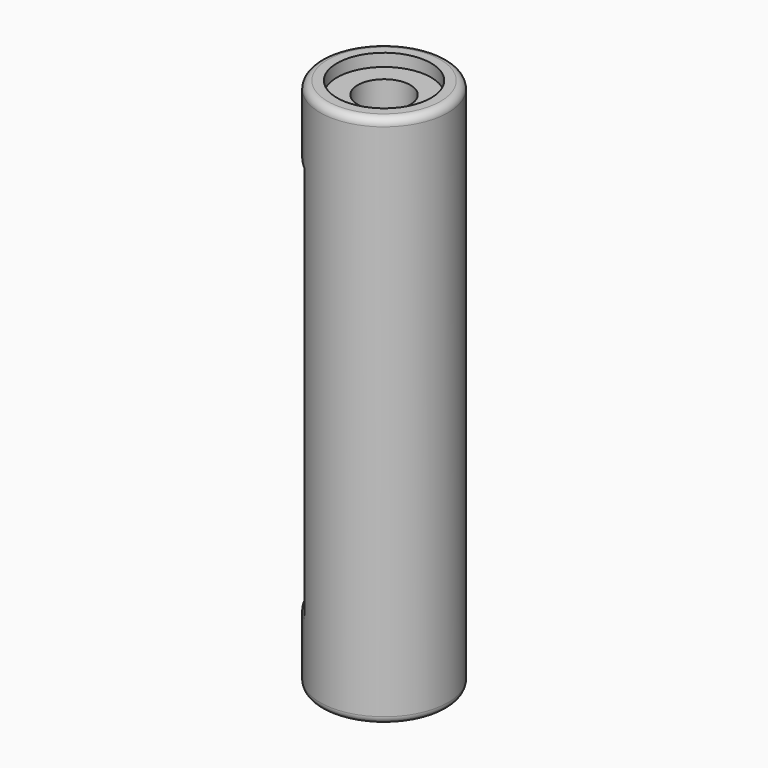
from build123d import *

# Parameters (mm, degrees)
F0_R          = 5.1
F0_R_2        = 2.1
F1_DEPTH      = 42.6
F2_R          = 3.5
F3_DEPTH      = 3.2
F4_R          = 3.75
F5_DEPTH      = 1
F6_W          = 6
F6_H          = 30.6
F7_DEPTH      = 25
F9_START      = -2.5
F8_R          = 3.1
F9_DEPTH      = 31.5
F10_T1_DEPTH  = 30.6
F10_T10_ANGLE = 105.7758372511
F10_T16_ANGLE = 105.7758372511
F10_T23_DEPTH = 34.3907560857
F10_T27_ANGLE = 105.7758372511
F10_T34_ANGLE = 105.7758372511
F10_T38_DEPTH = 34.3907560857
F10_T45_DEPTH = 34.3907560857
F10_T49_ANGLE = 105.7758372511
F10_T56_DEPTH = 34.3907560857
F10_T60_ANGLE = 105.7758372511


# Not quite as in the source:
# - a fillet or chamfer that OpenCascade refuses, or shapes differently, is made with other operations: its cross-section is extruded or revolved along the edge and cut away or added


with BuildPart() as f1:
    # F0 (on Top) → F1 (new body)
    with BuildSketch(Plane.XY):
        Circle(F0_R)
        Circle(F0_R_2, mode=Mode.SUBTRACT)
    extrude(amount=F1_DEPTH)

    # F2 (on face) → F3 (cut)
    with BuildSketch(Plane(origin=(0, 0, 0), x_dir=(1, 0, 0), z_dir=(0, 0, -1))):
        Circle(F2_R)
    extrude(amount=-F3_DEPTH, mode=Mode.SUBTRACT)

    # F4 (on face) → F5 (cut)
    with BuildSketch(Plane.XY.offset(42.6)):
        Circle(F4_R)
    extrude(amount=-F5_DEPTH, mode=Mode.SUBTRACT)

    # F6 (on Right) → F7 (cut)
    with BuildSketch(Plane.YZ):
        with Locations((0, 21.3)):
            Rectangle(F6_W, F6_H)
    extrude(amount=-F7_DEPTH, mode=Mode.SUBTRACT)

    # F8 (on face) → F9 (cut)
    with BuildSketch(Plane(origin=(0, 0, 3.2), x_dir=(1, 0, 0), z_dir=(0, 0, -1)).offset(F9_START)):
        Circle(F8_R)
    extrude(amount=-F9_DEPTH, mode=Mode.SUBTRACT)

    # F10: fillet of radius 0.6 on 6 edges, made by hand

    # F10_s2 → F10_t1 (cut)
    with BuildSketch(Plane.XY.offset(6)):
        with BuildLine():
            ThreePointArc((-3.06, 4.08), (-3.2692099788, 3.4102633404), (-2.7, 3))
            Line((-2.7, 3), (-4.1243181255, 3))
            ThreePointArc((-4.1243181255, 3), (-3.6325207132, 3.5797755891), (-3.06, 4.08))
        make_face()
        with BuildLine():
            ThreePointArc((-3.06, -4.08), (-3.2692099788, -3.4102633404), (-2.7, -3))
            Line((-2.7, -3), (-4.1243181255, -3))
            ThreePointArc((-4.1243181255, -3), (-3.6325207132, -3.5797755891), (-3.06, -4.08))
        make_face()
    extrude(amount=F10_T1_DEPTH, mode=Mode.SUBTRACT)

    # F10_s3 → F10_t4 (revolve, cut)
    with BuildSketch(Plane.XZ):
        with BuildLine():
            ThreePointArc((5.1, 42), (4.9242640687, 42.4242640687), (4.5, 42.6))
            Line((4.5, 42.6), (5.1, 42.6))
            Line((5.1, 42.6), (5.1, 42))
        make_face()
    revolve(axis=Axis((0, 0, 42.6), (0, 0, 1)), mode=Mode.SUBTRACT)

    # F10_s5 → F10_t6 (revolve, cut)
    with BuildSketch(Plane.XZ):
        with BuildLine():
            ThreePointArc((5.1, 0.6), (4.9242640687, 0.1757359313), (4.5, 0))
            Line((4.5, 0), (5.1, 0))
            Line((5.1, 0), (5.1, 0.6))
        make_face()
    revolve(axis=Axis((0, 0, 0), (0, 0, 1)), mode=Mode.SUBTRACT)


with BuildPart() as f10_tool8:
    # F10_s9 → F10_t10 (revolve)
    with BuildSketch(Plane(origin=(0, 0, 0), x_dir=(0, 0, 1), z_dir=(0.7974567188, -0.6033761527, 0))):
        with BuildLine():
            ThreePointArc((5.4, 5.1), (5.8242640687, 4.9242640687), (6, 4.5))
            Line((6, 4.5), (6, 5.1))
            Line((6, 5.1), (5.4, 5.1))
        make_face()
    revolve(axis=Axis((0, 0, 6), (0, 0, -1)), revolution_arc=F10_T10_ANGLE)

    split(bisect_by=Plane.XZ.offset(3), keep=Keep.BOTTOM)

    split(bisect_by=Plane.XZ.offset(-3), keep=Keep.TOP)


with BuildPart() as f1_1:
    add(f1.part)

    # F10_t7: cut F10_tool8
    add(f10_tool8.part, mode=Mode.SUBTRACT)


with BuildPart() as f10_tool14:
    # F10_s15 → F10_t16 (revolve)
    with BuildSketch(Plane(origin=(0, 0, 0), x_dir=(0, 0, 1), z_dir=(0.7974567188, -0.6033761527, 0))):
        with BuildLine():
            ThreePointArc((37.2, 5.1), (36.7757359313, 4.9242640687), (36.6, 4.5))
            Line((36.6, 4.5), (36.6, 5.1))
            Line((36.6, 5.1), (37.2, 5.1))
        make_face()
    revolve(axis=Axis((0, 0, 36.6), (0, 0, -1)), revolution_arc=F10_T16_ANGLE)

    split(bisect_by=Plane.XZ.offset(3), keep=Keep.BOTTOM)

    split(bisect_by=Plane.XZ.offset(-3), keep=Keep.TOP)


with BuildPart() as f1_2:
    add(f1_1.part)

    # F10_t13: cut F10_tool14
    add(f10_tool14.part, mode=Mode.SUBTRACT)


with BuildPart() as f10_tool21:
    # F10_s22 → F10_t23 (new body)
    with BuildSketch(Plane.XY.offset(36.6)):
        with BuildLine():
            ThreePointArc((-3.06, -4.08), (-3.2692099788, -3.4102633404), (-2.7, -3))
            Line((-2.7, -3), (-4.1243181255, -3))
            ThreePointArc((-4.1243181255, -3), (-3.6325207132, -3.5797755891), (-3.06, -4.08))
        make_face()
    extrude(amount=-F10_T23_DEPTH)

    split(bisect_by=Plane.XY.offset(6), keep=Keep.BOTTOM)


with BuildPart() as f10_tool25:
    # F10_s26 → F10_t27 (revolve)
    with BuildSketch(Plane(origin=(0, 0, 0), x_dir=(0, 0, 1), z_dir=(0.7974567188, -0.6033761527, 0))):
        with BuildLine():
            ThreePointArc((5.4, 5.1), (5.8242640687, 4.9242640687), (6, 4.5))
            Line((6, 4.5), (6, 5.1))
            Line((6, 5.1), (5.4, 5.1))
        make_face()
    revolve(axis=Axis((0, 0, 6), (0, 0, -1)), revolution_arc=F10_T27_ANGLE)

    split(bisect_by=Plane.XZ.offset(3), keep=Keep.TOP)


with BuildPart() as f10_tool21_1:
    add(f10_tool21.part)

    # F10_t29: intersect F10_tool25
    add(f10_tool25.part, mode=Mode.INTERSECT)


with BuildPart() as f1_3:
    add(f1_2.part)

    # F10_t19: cut F10_tool21
    add(f10_tool21_1.part, mode=Mode.SUBTRACT)


with BuildPart() as f10_tool32:
    # F10_s33 → F10_t34 (revolve)
    with BuildSketch(Plane(origin=(0, 0, 0), x_dir=(0, 0, 1), z_dir=(0.7974567188, -0.6033761527, 0))):
        with BuildLine():
            ThreePointArc((5.4, 5.1), (5.8242640687, 4.9242640687), (6, 4.5))
            Line((6, 4.5), (6, 5.1))
            Line((6, 5.1), (5.4, 5.1))
        make_face()
    revolve(axis=Axis((0, 0, 6), (0, 0, -1)), revolution_arc=F10_T34_ANGLE)

    split(bisect_by=Plane.XZ.offset(-3), keep=Keep.BOTTOM)


with BuildPart() as f10_tool36:
    # F10_s37 → F10_t38 (new body)
    with BuildSketch(Plane.XY.offset(36.6)):
        with BuildLine():
            ThreePointArc((-3.06, 4.08), (-3.2692099788, 3.4102633404), (-2.7, 3))
            Line((-2.7, 3), (-4.1243181255, 3))
            ThreePointArc((-4.1243181255, 3), (-3.6325207132, 3.5797755891), (-3.06, 4.08))
        make_face()
    extrude(amount=-F10_T38_DEPTH)

    split(bisect_by=Plane.XY.offset(6), keep=Keep.BOTTOM)


with BuildPart() as f10_tool32_1:
    add(f10_tool32.part)

    # F10_t40: intersect F10_tool36
    add(f10_tool36.part, mode=Mode.INTERSECT)


with BuildPart() as f1_4:
    add(f1_3.part)

    # F10_t30: cut F10_tool32
    add(f10_tool32_1.part, mode=Mode.SUBTRACT)


with BuildPart() as f10_tool43:
    # F10_s44 → F10_t45 (new body)
    with BuildSketch(Plane.XY.offset(40.3907560857)):
        with BuildLine():
            ThreePointArc((-3.06, 4.08), (-3.2692099788, 3.4102633404), (-2.7, 3))
            Line((-2.7, 3), (-4.1243181255, 3))
            ThreePointArc((-4.1243181255, 3), (-3.6325207132, 3.5797755891), (-3.06, 4.08))
        make_face()
    extrude(amount=-F10_T45_DEPTH)

    split(bisect_by=Plane.XY.offset(36.6), keep=Keep.TOP)


with BuildPart() as f10_tool47:
    # F10_s48 → F10_t49 (revolve)
    with BuildSketch(Plane(origin=(0, 0, 0), x_dir=(0, 0, 1), z_dir=(0.7974567188, -0.6033761527, 0))):
        with BuildLine():
            ThreePointArc((37.2, 5.1), (36.7757359313, 4.9242640687), (36.6, 4.5))
            Line((36.6, 4.5), (36.6, 5.1))
            Line((36.6, 5.1), (37.2, 5.1))
        make_face()
    revolve(axis=Axis((0, 0, 36.6), (0, 0, -1)), revolution_arc=F10_T49_ANGLE)

    split(bisect_by=Plane.XZ.offset(-3), keep=Keep.BOTTOM)


with BuildPart() as f10_tool43_1:
    add(f10_tool43.part)

    # F10_t51: intersect F10_tool47
    add(f10_tool47.part, mode=Mode.INTERSECT)


with BuildPart() as f1_5:
    add(f1_4.part)

    # F10_t41: cut F10_tool43
    add(f10_tool43_1.part, mode=Mode.SUBTRACT)


with BuildPart() as f10_tool54:
    # F10_s55 → F10_t56 (new body)
    with BuildSketch(Plane.XY.offset(40.3907560857)):
        with BuildLine():
            ThreePointArc((-3.06, -4.08), (-3.2692099788, -3.4102633404), (-2.7, -3))
            Line((-2.7, -3), (-4.1243181255, -3))
            ThreePointArc((-4.1243181255, -3), (-3.6325207132, -3.5797755891), (-3.06, -4.08))
        make_face()
    extrude(amount=-F10_T56_DEPTH)

    split(bisect_by=Plane.XY.offset(36.6), keep=Keep.TOP)


with BuildPart() as f10_tool58:
    # F10_s59 → F10_t60 (revolve)
    with BuildSketch(Plane(origin=(0, 0, 0), x_dir=(0, 0, 1), z_dir=(0.7974567188, -0.6033761527, 0))):
        with BuildLine():
            ThreePointArc((37.2, 5.1), (36.7757359313, 4.9242640687), (36.6, 4.5))
            Line((36.6, 4.5), (36.6, 5.1))
            Line((36.6, 5.1), (37.2, 5.1))
        make_face()
    revolve(axis=Axis((0, 0, 36.6), (0, 0, -1)), revolution_arc=F10_T60_ANGLE)

    split(bisect_by=Plane.XZ.offset(3), keep=Keep.TOP)


with BuildPart() as f10_tool54_1:
    add(f10_tool54.part)

    # F10_t62: intersect F10_tool58
    add(f10_tool58.part, mode=Mode.INTERSECT)


with BuildPart() as f1_6:
    add(f1_5.part)

    # F10_t52: cut F10_tool54
    add(f10_tool54_1.part, mode=Mode.SUBTRACT)


solid = f1_6.part
